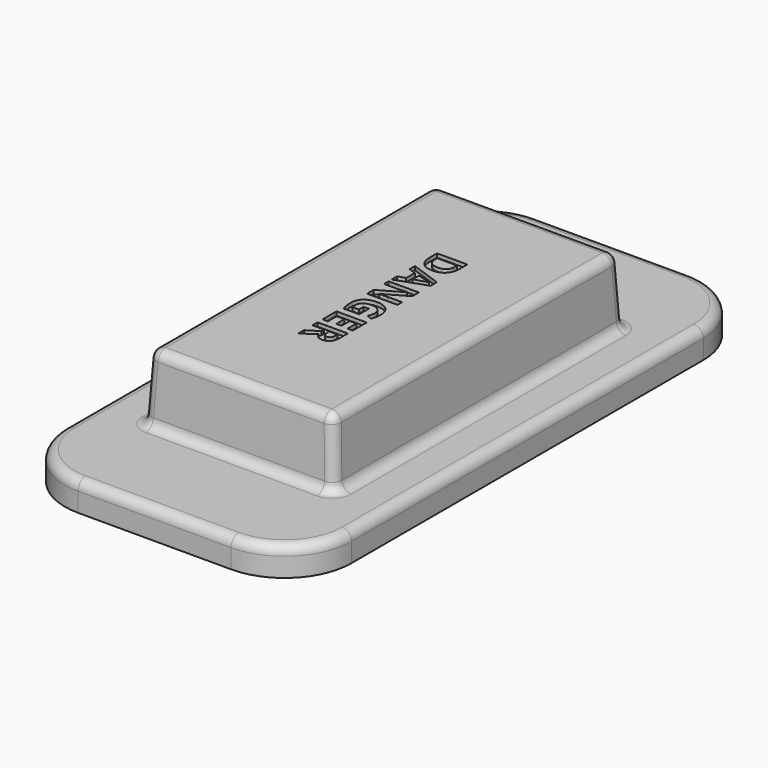
from build123d import *

# Parameters (mm, degrees)
F0_W         = 30
F0_H         = 60
F1_DEPTH     = 3
F2_W         = 20
F2_H         = 38
F3_DEPTH     = 7
F3_TAPER     = 3
F4_W         = 17
F4_H         = 35
F6_DEPTH     = 6
F6_TAPER     = -3
F5_R         = 4.25
F7_DEPTH     = 2
F8_TEXT_SIZE = 4.4311332102
F9_DEPTH     = 0.4
F10_R        = 7
F11_R        = 1


# Not quite as in the source:
# - Text() gives the source's letters only with a copy of the font that has no kerning and outlines rounded to 1/6400 em; it was checked with that copy


with BuildPart() as f1:
    # F0 (on Top) → F1 (new body)
    with BuildSketch(Plane.XY):
        Rectangle(F0_W, F0_H)
    extrude(amount=F1_DEPTH)

    # F2 (on face) → F3 (join)
    with BuildSketch(Plane.XY.offset(3)):
        Rectangle(F2_W, F2_H)
    extrude(amount=F3_DEPTH, taper=F3_TAPER)

    # F4 (on face) → F6 (cut)
    with BuildSketch(Plane.XY):
        Rectangle(F4_W, F4_H)
    extrude(amount=F6_DEPTH, taper=F6_TAPER, mode=Mode.SUBTRACT)

    # F5 (on face) → F7 (cut)
    with BuildSketch(Plane.XY):
        with Locations((0, -24.5)):
            Circle(F5_R)
        with Locations((0, 24.5)):
            Circle(F5_R)
    extrude(amount=F7_DEPTH, mode=Mode.SUBTRACT)

    # F8 (on face) → F9 (cut)
    with BuildSketch(Plane.XY.offset(10)):
        with Locations(Location((-1.7882763641, 9.5710428432), (0, 0, -90))):
            Text('DANGER', F8_TEXT_SIZE, font='Open Sans', font_style=FontStyle.BOLD, text_align=(TextAlign.LEFT, TextAlign.BOTTOM))
    extrude(amount=-F9_DEPTH, mode=Mode.SUBTRACT)

    # F10
    f10_edges = [f1.edges().sort_by_distance(p)[0] for p in [
        (-15, 30, 1.5),
        (15, 30, 1.5),
        (-15, -30, 1.5),
        (15, -30, 1.5),
    ]]
    fillet(f10_edges, radius=F10_R)

    # F11
    f11_edges = [f1.edges().sort_by_distance(p)[0] for p in [
        (-9.816573, 18.816573, 6.5),
        (-9.816573, -18.816573, 6.5),
        (9.816573, -18.816573, 6.5),
        (9.816573, 18.816573, 6.5),
        (9.633146, 0, 10),
        (0, -18.633146, 10),
        (-9.633146, 0, 10),
        (0, 18.633146, 10),
        (-10, 0, 3),
        (-15, 0, 3),
        (0, 30, 3),
        (12.949747, 27.949747, 3),
        (-12.949747, 27.949747, 3),
        (15, 0, 3),
        (12.949747, -27.949747, 3),
        (-12.949747, -27.949747, 3),
        (0, -30, 3),
        (0, 19, 3),
        (0, -19, 3),
        (10, 0, 3),
    ]]
    fillet(f11_edges, radius=F11_R)


solid = f1.part
